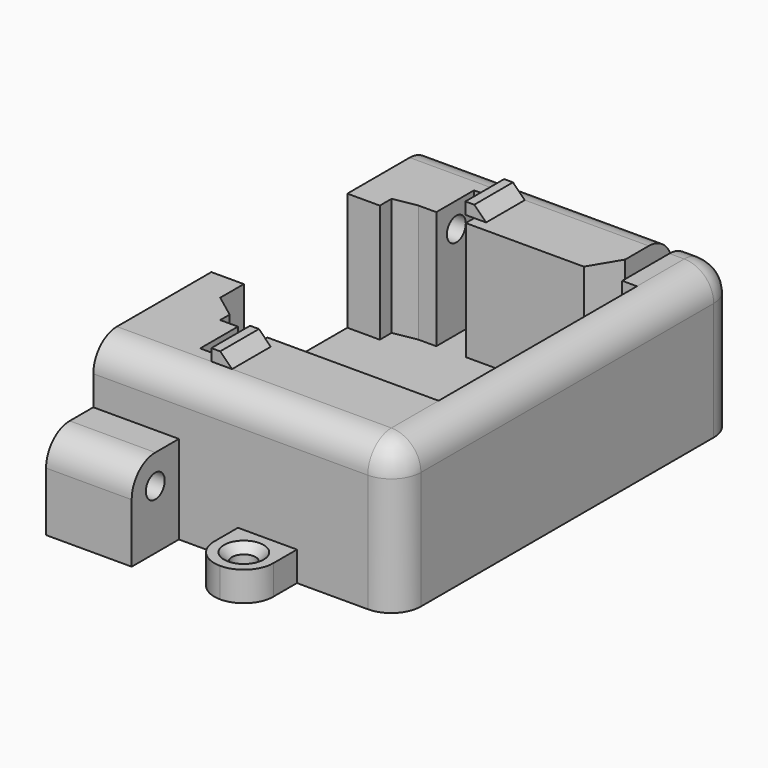
from build123d import *

# Parameters (mm, degrees)
F1_DEPTH        = 20
F3_DEPTH        = 5
F5_W            = 10
F5_H            = 15
F6_DEPTH        = 10
F7_R            = 5
F8_W            = 10
F8_H            = 15
F9_DEPTH        = 10
F10_R           = 5
F12_D           = 4
F14_D           = 4
F14_DEPTH       = 17
F14_TIP         = 1.2017212381
F15_R           = 4.99999
F16_T1_DEPTH    = 25
F16_T3_DEPTH    = 15.00001
F16_T5_DEPTH    = 32.50001
F16_T8_ANGLE    = 90
F16_T10_ANGLE   = 90
F17_W           = 2
F17_H           = 8.2
F18_DEPTH       = 2
F19_W           = 8.2
F19_H           = 2
F20_DEPTH       = 1.5
F21_SIZE        = 1.99999
F22_DEPTH       = 4.5
F23_W           = 10
F23_H           = 10
F24_DEPTH       = 5
F25_R           = 4.99999
F27_D           = 4
F27_CSINK_D     = 6.72
F27_CSINK_ANGLE = 90


# Not quite as in the source:
# - a fillet or chamfer that OpenCascade refuses, or shapes differently, is made with other operations: its cross-section is extruded or revolved along the edge and cut away or added
# - a fillet or chamfer is up to 0.001 mm smaller than in the source, because OpenCascade refuses the exact size


with BuildPart() as f1:
    # F0 (on Top) → F1 (new body)
    with BuildSketch(Plane.XY):
        Polygon((-23.5, -36), (23.5, -36), (23.5, 36), (16, 36), (16, 21), (18.5, 21), (18.5, -21), (-10.5, -21), (-10.5, -29), (-15.5, -29), (-15.5, -21), (-18.5, -21), (-18.5, -19), (-22.5, -16), (-22.5, -11), (-23.5, -11), align=None)
    extrude(amount=F1_DEPTH)


with BuildPart() as f1b:
    # F0 (on Top) → F1, piece 2 (new body)
    with BuildSketch(Plane.XY):
        Polygon((12.5, 26), (12.5, 36), (-23.5, 36), (-23.5, 17.7946920772), (-22.5, 17.7946920772), (-22.5, 20.2946920772), (-18.5, 21), (-15.5, 21), (-15.5, 29), (-10.5, 29), (-10.5, 21), (9.5, 21), align=None)
    extrude(amount=F1_DEPTH)


with BuildPart() as f3:
    # F2 (on face) → F3 (new body)
    with BuildSketch(Plane.XY):
        Polygon((23.5, -36), (23.5, 36), (16, 36), (16, 21), (18.5, 21), (18.5, -21), (-10.5, -21), (-15.5, -21), (-18.5, -21), (-18.5, -19), (-22.5, -16), (-22.5, -11), (-22.5, 0), (-22.5, 17.7946920772), (-22.5, 20.2946920772), (-18.5, 21), (-15.5, 21), (-10.5, 21), (9.5, 21), (12.5, 26), (12.5, 36), (-23.5, 36), (-23.5, -36), align=None)
        Polygon((16, 21), (16, 36), (12.5, 36), (12.5, 26), (9.5, 21), (-10.5, 21), (-15.5, 21), (-18.5, 21), (-22.5, 20.2946920772), (-22.5, 17.7946920772), (-22.5, 0), (-22.5, -11), (-22.5, -16), (-18.5, -19), (-18.5, -21), (-15.5, -21), (-10.5, -21), (18.5, -21), (18.5, 21), align=None)
    extrude(amount=-F3_DEPTH)


with BuildPart() as f1b_1:
    add(f1b.part)

    # F4: union F3, F1
    add(f3.part)
    add(f1.part)

    # F5 (on face) → F6 (join)
    with BuildSketch(Plane.XZ.offset(36)):
        with Locations((-18.5, 2.5)):
            Rectangle(F5_W, F5_H)
    extrude(amount=F6_DEPTH)

    # F7
    f7_edges = [f1b_1.edges().sort_by_distance(p)[0] for p in [
        (-18.5, -46, 10),
    ]]
    fillet(f7_edges, radius=F7_R)

    # F8 (on face) → F9 (join)
    with BuildSketch(Plane(origin=(0, 36, 0), x_dir=(-1, 0, 0), z_dir=(0, 1, 0))):
        with Locations((18.5, 2.5)):
            Rectangle(F8_W, F8_H)
    extrude(amount=F9_DEPTH)

    # F10
    f10_edges = [f1b_1.edges().sort_by_distance(p)[0] for p in [
        (-18.5, 46, 10),
    ]]
    fillet(f10_edges, radius=F10_R)

    # F12 (through all)
    with Locations(Plane(origin=(-23.5, 0, 0), x_dir=(0, -1, 0), z_dir=(-1, 0, 0))):
        with Locations((-41, 5), (41, 5)):
            Hole(F12_D / 2)

    # F14
    with Locations(Plane(origin=(-23.5, 0, 0), x_dir=(0, -1, 0), z_dir=(-1, 0, 0))):
        with Locations((-25.25, 15.75), (25.25, 15.75)):
            Hole(F14_D / 2, depth=F14_DEPTH)
            with Locations((0, 0, -(F14_DEPTH + F14_TIP / 2))):  # 118° drill point
                Cone(0, F14_D / 2, F14_TIP, mode=Mode.SUBTRACT)

    # F15 (radius 5 in the source; OpenCascade refuses exactly that, so slightly less here)
    f15_edges = [f1b_1.edges().sort_by_distance(p)[0] for p in [
        (-5.5, 36, 20),
        (0, -36, 20),
        (23.5, 0, 20),
    ]]
    fillet(f15_edges, radius=F15_R)

    # F16: fillet of radius 5 on 2 edges, made by hand

    # F16_s2 → F16_t1 (cut)
    with BuildSketch(Plane.XY.offset(-5)):
        with BuildLine():
            ThreePointArc((18.5, -36), (22.0355339059, -34.5355339059), (23.5, -31))
            Line((23.5, -31), (23.6, -31))
            Line((23.6, -31), (23.6, -36.1))
            Line((23.6, -36.1), (18.5, -36.1))
            Line((18.5, -36.1), (18.5, -36))
        make_face()
    extrude(amount=F16_T1_DEPTH, mode=Mode.SUBTRACT)

    # F16_s4 → F16_t3 (cut)
    with BuildSketch(Plane.YZ.offset(16)):
        with BuildLine():
            ThreePointArc((36, 15), (34.5355339059, 18.5355339059), (31, 20))
            Line((31, 20), (31, 20.1))
            Line((31, 20.1), (36.1, 20.1))
            Line((36.1, 20.1), (36.1, 15))
            Line((36.1, 15), (36, 15))
        make_face()
    extrude(amount=F16_T3_DEPTH, mode=Mode.SUBTRACT)

    # F16_s6 → F16_t5 (cut)
    with BuildSketch(Plane.XY.offset(-5)):
        with BuildLine():
            ThreePointArc((18.5, 36), (22.0355339059, 34.5355339059), (23.5, 31))
            Line((23.5, 31), (23.6, 31))
            Line((23.6, 31), (23.6, 36.1))
            Line((23.6, 36.1), (18.5, 36.1))
            Line((18.5, 36.1), (18.5, 36))
        make_face()
    extrude(amount=F16_T5_DEPTH, mode=Mode.SUBTRACT)

    # F16_s7 → F16_t8 (revolve, cut)
    with BuildSketch(Plane.YZ.offset(18.5)):
        with BuildLine():
            ThreePointArc((-31.00001, 20), (-34.5355368349, 18.5355368349), (-36, 15.00001))
            Line((-36, 15.00001), (-36, 20))
            Line((-36, 20), (-31.00001, 20))
        make_face()
    revolve(axis=Axis((18.5, -31, 20), (0, 0, 1)), revolution_arc=F16_T8_ANGLE, mode=Mode.SUBTRACT)

    # F16_s9 → F16_t10 (revolve, cut)
    with BuildSketch(Plane.YZ.offset(18.50001)):
        with BuildLine():
            ThreePointArc((36, 15.00001), (34.5355303704, 18.5355374415), (31, 20))
            Line((31, 20), (31, 20.1))
            Line((31, 20.1), (36.1, 20.1))
            Line((36.1, 20.1), (36.1, 15.00001))
            Line((36.1, 15.00001), (36, 15.00001))
        make_face()
    revolve(axis=Axis((18.50001, 36, 15.00001), (0, 1, 0)), revolution_arc=F16_T10_ANGLE, mode=Mode.SUBTRACT)

    # F17 (on face) → F18 (join)
    with BuildSketch(Plane.XY.offset(20)):
        Polygon((-8.5, -22.8), (-10.5, -22.8), (-10.5, -29), (-10.5, -31), (-8.5, -31), align=None)
        with Locations((-9.5, 26.9)):
            Rectangle(F17_W, F17_H)
    extrude(amount=F18_DEPTH)

    # F19 (on face) → F20 (join)
    with BuildSketch(Plane(origin=(-10.5, 0, 0), x_dir=(0, -1, 0), z_dir=(-1, 0, 0))):
        Polygon((-22.8, 22), (-31, 22), (-31, 20), (-29, 20), (-22.8, 20), align=None)
        with Locations((26.9, 21)):
            Rectangle(F19_W, F19_H)
    extrude(amount=F20_DEPTH)

    # F21 (size 2 in the source; OpenCascade refuses exactly that, so slightly less here)
    f21_edges = [f1b_1.edges().sort_by_distance(p)[0] for p in [
        (-8.5, -26.9, 22),
        (-8.5, 26.9, 22),
    ]]
    chamfer(f21_edges, length=F21_SIZE)

    # F22 (add): a face of the model
    f22_faces = [f1b_1.faces().sort_by_distance(p)[0] for p in [
        (-23.5, 35.0466375296, 12.500005),
    ]]
    extrude(f22_faces, amount=F22_DEPTH)

    # F23 (on face) → F24 (join)
    with BuildSketch(Plane(origin=(0, 0, -5), x_dir=(1, 0, 0), z_dir=(0, 0, -1))):
        with Locations((1.5, -41)):
            Rectangle(F23_W, F23_H)
        with Locations((1.5, 41)):
            Rectangle(F23_W, F23_H)
    extrude(amount=-F24_DEPTH)

    # F25 (radius 5 in the source; OpenCascade refuses exactly that, so slightly less here)
    f25_edges = [f1b_1.edges().sort_by_distance(p)[0] for p in [
        (6.5, -46, -2.5),
        (-3.5, -46, -2.5),
        (6.5, 46, -2.5),
        (-3.5, 46, -2.5),
    ]]
    fillet(f25_edges, radius=F25_R)

    # F27 (through all)
    with Locations(Plane.XY):
        with Locations((1.5, -41), (1.5, 41)):
            CounterSinkHole(F27_D / 2, F27_CSINK_D / 2, counter_sink_angle=F27_CSINK_ANGLE)


solid = f1b_1.part
